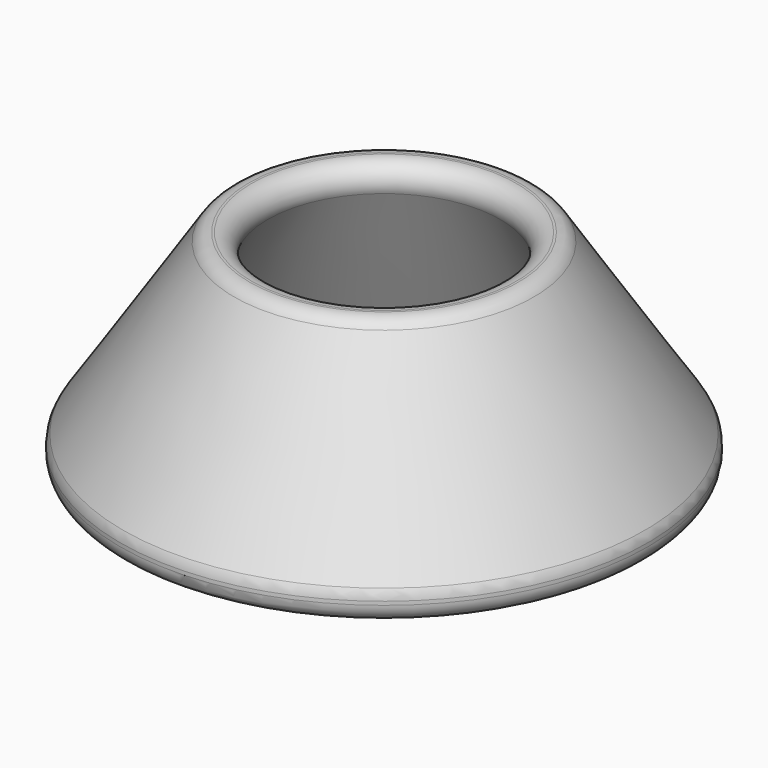
from build123d import *

# Parameters (mm, degrees)
F5_R = 2.5


# Not quite as in the source:
# - the program builds the solid bodies; features that only make, move or delete a surface that nothing else refers to are left out


with BuildPart() as f4:
    # F3 (on Front) → F4 (revolve)
    with BuildSketch(Plane.XZ):
        Polygon((-36.259230652, 20.2593781938), (-28.4696114573, 20.2593781938), (-14.1603897064, 49), (-19.8540338413, 49), (-36.259230652, 24), align=None)
    revolve(axis=Axis((0, 0, 18.828805536), (0, 0, 1)))

    # F5
    f5_edges = [f4.edges().sort_by_distance(p)[0] for p in [
        (19.854034, 0, 49),
        (14.16039, 0, 49),
        (36.259231, 0, 24),
        (36.259231, 0, 20.259378),
        (28.469611, 0, 20.259378),
    ]]
    fillet(f5_edges, radius=F5_R)


solid = f4.part
